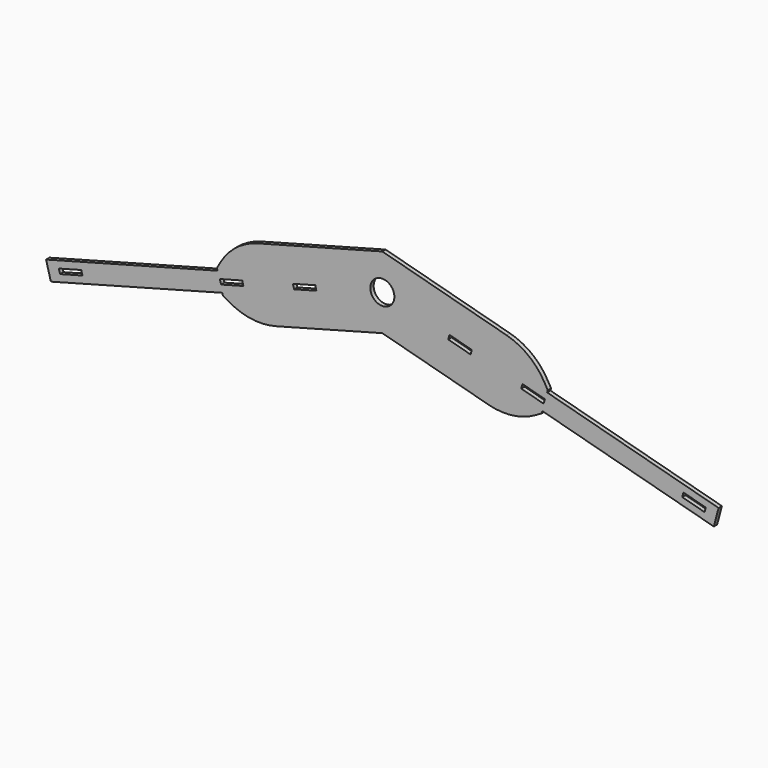
from build123d import *

# Parameters (mm, degrees)
F0_R     = 9.906
F1_DEPTH = 3.429


# Not quite as in the source:
# - ends of sketch curves that miss each other by under 0.0002 mm in the source are joined


with BuildPart() as f1:
    # F0 (on Front) → F1 (new body)
    with BuildSketch(Plane.XZ):
        with BuildLine():
            ThreePointArc((121.3266326526, 283.5242564606), (141.1053673826, 282.2278907762), (159.8746336835, 288.5991978658))
            Line((159.8746336835, 288.5991978658), (164.9830584, 291.548566))
            Line((164.9830584, 291.548566), (165.4761232, 293.3886436))
            Line((165.4761232, 293.3886436), (306.5495774, 255.588135))
            Line((306.5495774, 255.588135), (310.4939942, 270.308832))
            Line((310.4939942, 270.308832), (169.4205146, 308.109366))
            Line((169.4205146, 308.109366), (169.9135794, 309.9494436))
            Line((169.9135794, 309.9494436), (166.9642076, 315.0578916))
            ThreePointArc((166.9642076, 315.0578916), (153.8951945869, 329.9602399108), (136.1181216974, 338.7269230379))
            Line((136.1181216974, 338.7269230379), (33.7705954, 366.1508552))
            Line((33.7705954, 366.1508552), (-68.5769266, 338.726907))
            ThreePointArc((-68.5769266, 338.726907), (-86.3539881192, 329.9602324429), (-99.4229877342, 315.0578894835))
            Line((-99.4229877342, 315.0578894835), (-102.3723632, 309.9494436))
            Line((-102.3723632, 309.9494436), (-101.8792984, 308.109366))
            Line((-101.8792984, 308.109366), (-242.952778, 270.308832))
            Line((-242.952778, 270.308832), (-239.0083612, 255.588135))
            Line((-239.0083612, 255.588135), (-97.934907, 293.3886436))
            Line((-97.934907, 293.3886436), (-97.4418676, 291.548566))
            Line((-97.4418676, 291.548566), (-92.3334196, 288.5991942))
            ThreePointArc((-92.3334196, 288.5991942), (-73.5641511826, 282.2278907762), (-53.7854164526, 283.5242564606))
            Line((-53.7854164526, 283.5242564606), (33.7705954, 306.9848318))
            Line((33.7705954, 306.9848318), (121.3266326526, 283.5242564606))
        make_face()
        Polygon((-232.4312598, 267.2114544), (-214.0303568, 272.1419754), (-213.044278, 268.4617948), (-231.4451556, 263.5312992), align=None, mode=Mode.SUBTRACT)
        Polygon((-99.9448598, 302.7110786), (-81.5439822, 307.6415996), (-80.557878, 303.961419), (-98.9587556, 299.030898), align=None, mode=Mode.SUBTRACT)
        Polygon((280.5854688, 268.4617948), (281.571573, 272.1419754), (299.972476, 267.2114544), (298.9863718, 263.5312992), align=None, mode=Mode.SUBTRACT)
        Polygon((167.486076, 302.7110786), (166.4999718, 299.030898), (148.0990942, 303.961419), (149.0851984, 307.6415996), align=None, mode=Mode.SUBTRACT)
        Polygon((-39.8353026, 318.8173964), (-21.434425, 323.747892), (-20.4483208, 320.0677114), (-38.8491984, 315.1372158), align=None, mode=Mode.SUBTRACT)
        with Locations((33.7705954, 336.5678308)):
            Circle(F0_R, mode=Mode.SUBTRACT)
        Polygon((87.989537, 320.0677114), (88.9756158, 323.747892), (107.3765188, 318.8173964), (106.3904146, 315.1372158), align=None, mode=Mode.SUBTRACT)
    extrude(amount=F1_DEPTH)


solid = f1.part
